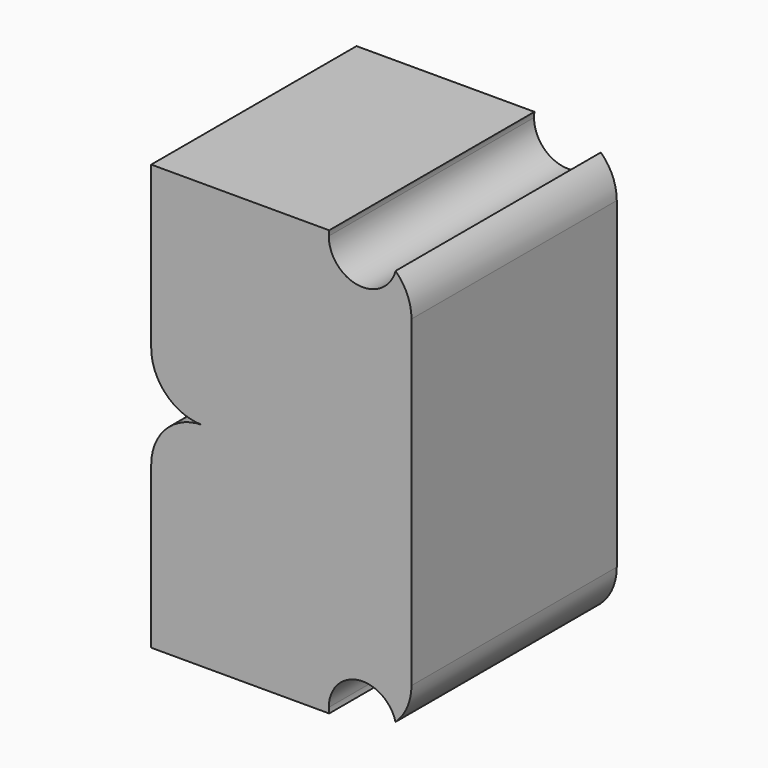
from build123d import *

# Parameters (mm, degrees)
F1_DEPTH = 25
F4_DEPTH = 25


# Not quite as in the source:
# - a pattern or mirror of a feature is missing from the dataset's text; its kind, count and spacing are read off the source's solid


with BuildPart() as f1:
    # F0 (on Front) → F1 (new body)
    with BuildSketch(Plane.XZ):
        with BuildLine():
            ThreePointArc((0, 5), (1.4644660941, 1.4644660941), (5, 0))
            Line((5, 0), (25.3563662991, 0))
            Line((25.3563662991, 0), (25.3563662991, 15.7199426368))
            ThreePointArc((25.3563662991, 15.7199426368), (23.891900205, 19.2554765427), (20.3563662991, 20.7199426368))
            Line((20.3563662991, 20.7199426368), (0, 20.7199426368))
            Line((0, 20.7199426368), (0, 5))
        make_face()
    extrude(amount=F1_DEPTH)

    # F2: F1 across face


with BuildPart() as f1_1:
    add(f1.part)
    add(f1.part.mirror(Plane(origin=(15.1781831495, -12.5, 0), x_dir=(1, 0, 0), z_dir=(0, 0, -1))))

    # F3 (on face) → F4 (cut)
    with BuildSketch(Plane(origin=(0, 0, 0), x_dir=(-1, 0, 0), z_dir=(0, 1, 0))):
        with BuildLine():
            Line((-20.3563662991, 20.7199426368), (-17.3368447248, 20.7199426368))
            ThreePointArc((-17.3368447248, 20.7199426368), (-21.2996072768, 23.4502367244), (-23.8041703997, 19.34108153))
            ThreePointArc((-23.8041703997, 19.34108153), (-22.2130172536, 20.3624470507), (-20.3563662991, 20.7199426368))
        make_face()
        with BuildLine():
            ThreePointArc((-23.8041703997, 19.34108153), (-20.1700051206, 16.929235893), (-17.2975812754, 20.2115122229))
            ThreePointArc((-17.2975812754, 20.2115122229), (-17.3074117289, 20.4664843313), (-17.3368447248, 20.7199426368))
            Line((-17.3368447248, 20.7199426368), (-20.3563662991, 20.7199426368))
            ThreePointArc((-20.3563662991, 20.7199426368), (-22.2130172536, 20.3624470507), (-23.8041703997, 19.34108153))
        make_face()
    f4 = extrude(amount=-F4_DEPTH, mode=Mode.SUBTRACT)

    # F4_copies: F4 across plane
    add(f4.mirror(Plane(origin=(0, 0, 0), x_dir=(-1, 0, 0), z_dir=(0, 0, -1))), mode=Mode.SUBTRACT)


solid = f1_1.part
